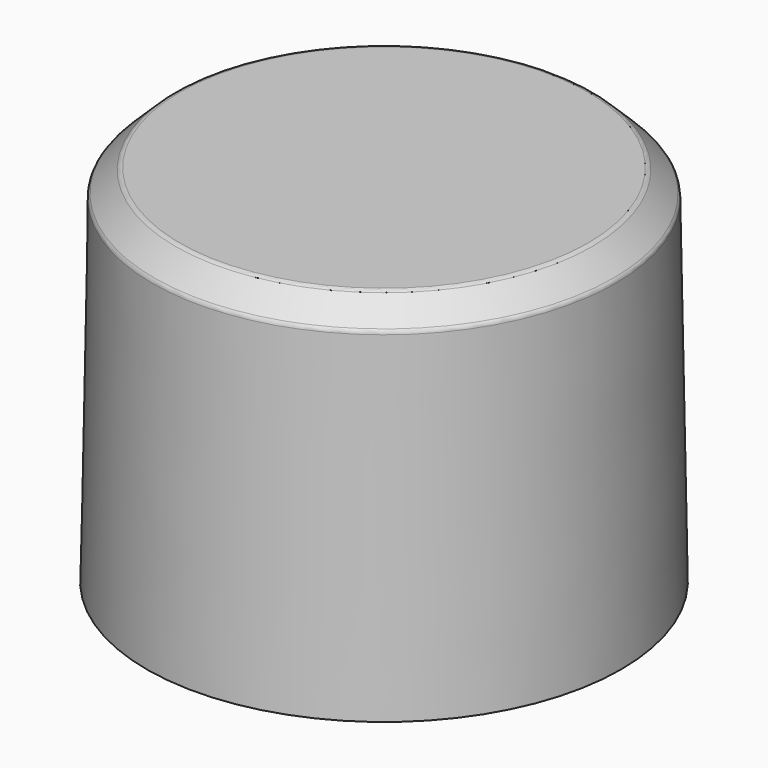
from build123d import *

# Parameters (mm, degrees)
F0_R     = 4
F1_DEPTH = 6
F3_SIZE  = 0.4
F4_R     = 0.1


# Not quite as in the source:
# - a fillet or chamfer that OpenCascade refuses, or shapes differently, is made with other operations: its cross-section is extruded or revolved along the edge and cut away or added


with BuildPart() as f1:
    # F0 (on Top) → F1 (new body)
    with BuildSketch(Plane.XY):
        Circle(F0_R)
    extrude(amount=F1_DEPTH)

    # F2: chamfer of 0.2 x 11.4579923262 on 1 edges, made by hand

    # F2_s1 → F2_t2 (revolve, cut)
    with BuildSketch(Plane.XZ):
        Polygon((4, -5.4579923262), (3.8, 6), (4, 6), align=None)
    revolve(axis=Axis((0, 0, 6), (0, 0, 1)), mode=Mode.SUBTRACT)

    # F3
    f3_edges = [f1.edges().sort_by_distance(p)[0] for p in [
        (-3.8, 0, 6),
    ]]
    chamfer(f3_edges, length=F3_SIZE)

    # F4
    f4_edges = [f1.edges().sort_by_distance(p)[0] for p in [
        (-3.4, 0, 6),
        (-3.806981, 0, 5.600061),
    ]]
    fillet(f4_edges, radius=F4_R)


solid = f1.part
